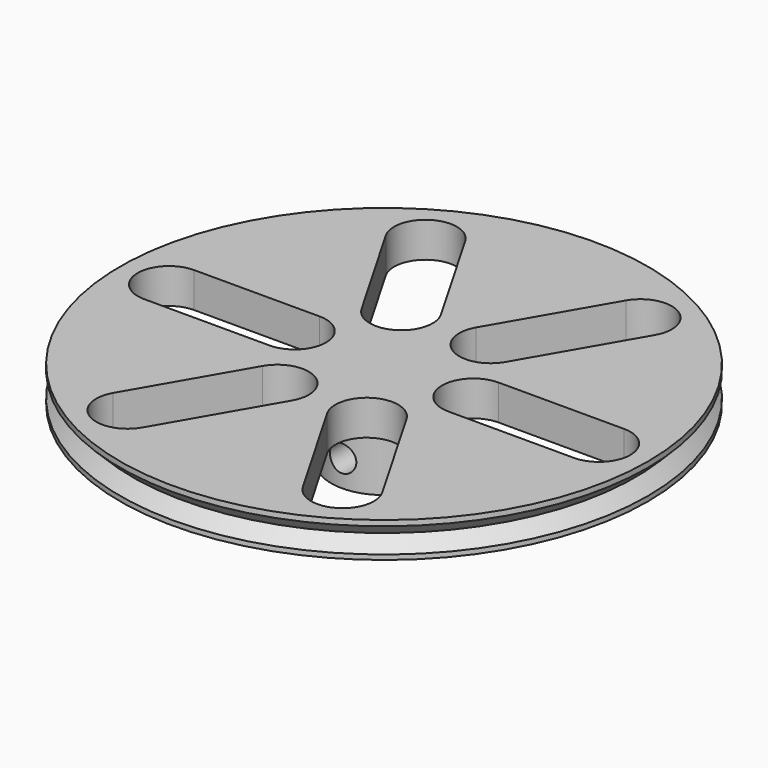
from build123d import *

# Parameters (mm, degrees)
F0_R             = 30
F0_R_2           = 6
F1_DEPTH         = 4
F2_DEPTH         = 6
F3_R             = 1.5
F4_DEPTH         = 13
F5_W             = 4.6
F5_H             = 3
F6_DEPTH         = 9.4
F10_W            = 14.2674595118
F10_H            = 7.1337288246
F11_DEPTH        = 12.5
F11_COPIES_COUNT = 6


# Not quite as in the source:
# - a pattern or mirror of a feature is missing from the dataset's text; its kind, count and spacing are read off the source's solid


with BuildPart() as f1:
    # F0 (on Top) → F1 (new body)
    with BuildSketch(Plane.XY):
        Circle(F0_R)
        Circle(F0_R_2, mode=Mode.SUBTRACT)
        Circle(F0_R_2)
    extrude(amount=F1_DEPTH)

    # F0 (on Top) → F2 (join)
    with BuildSketch(Plane.XY):
        Circle(F0_R_2)
    extrude(amount=-F2_DEPTH)

    # F3 (on Front) → F4 (cut, symmetric)
    with BuildSketch(Plane.XZ):
        with Locations((0, -3)):
            Circle(F3_R)
    extrude(amount=F4_DEPTH, both=True, mode=Mode.SUBTRACT)

    # F5 (on face) → F6 (cut)
    with BuildSketch(Plane(origin=(0, 0, -6), x_dir=(1, 0, 0), z_dir=(0, 0, -1))):
        with BuildLine():
            ThreePointArc((2.3, -1.5), (2.7459060435, 0), (2.3, 1.5))
            Line((2.3, 1.5), (2.3, -1.5))
        make_face()
        Rectangle(F5_W, F5_H)
        with BuildLine():
            Line((-2.3, -1.5), (-2.3, 1.5))
            ThreePointArc((-2.3, 1.5), (-2.7459060435, 0), (-2.3, -1.5))
        make_face()
    extrude(amount=-F6_DEPTH, mode=Mode.SUBTRACT)

    # F7 (on Front) → F9 (revolve, cut)
    with BuildSketch(Plane.XZ):
        Polygon((-30, 3.3777931239), (-30, 0.5493659992), (-28.5857864376, 1.9635795616), align=None)
    revolve(axis=Axis((0, 0, -3.6810841411), (0, 0, 1)), mode=Mode.SUBTRACT)

    # F10 (on Top) → F11 (cut, symmetric)
    with BuildSketch(Plane.XY):
        with Locations((-17.2992926091, 0)):
            Rectangle(F10_W, F10_H)
        with BuildLine():
            ThreePointArc((-24.433022365, 3.5668644123), (-27.9998867773, 0), (-24.433022365, -3.5668644123))
            Line((-24.433022365, -3.5668644123), (-24.433022365, 3.5668644123))
        make_face()
        with BuildLine():
            Line((-10.1655628532, 3.5668644123), (-10.1655628532, -3.5668644123))
            ThreePointArc((-10.1655628532, -3.5668644123), (-6.5986984409, 0), (-10.1655628532, 3.5668644123))
        make_face()
    f11 = extrude(amount=F11_DEPTH, both=True, mode=Mode.SUBTRACT)

    # F11_copies: F11 ×6 about axis
    f11_copies_axis = Axis((0, 0, 0), (0, 0, 1))
    for i in range(1, F11_COPIES_COUNT):
        add(f11.rotate(f11_copies_axis, i * 360 / F11_COPIES_COUNT), mode=Mode.SUBTRACT)


solid = f1.part
